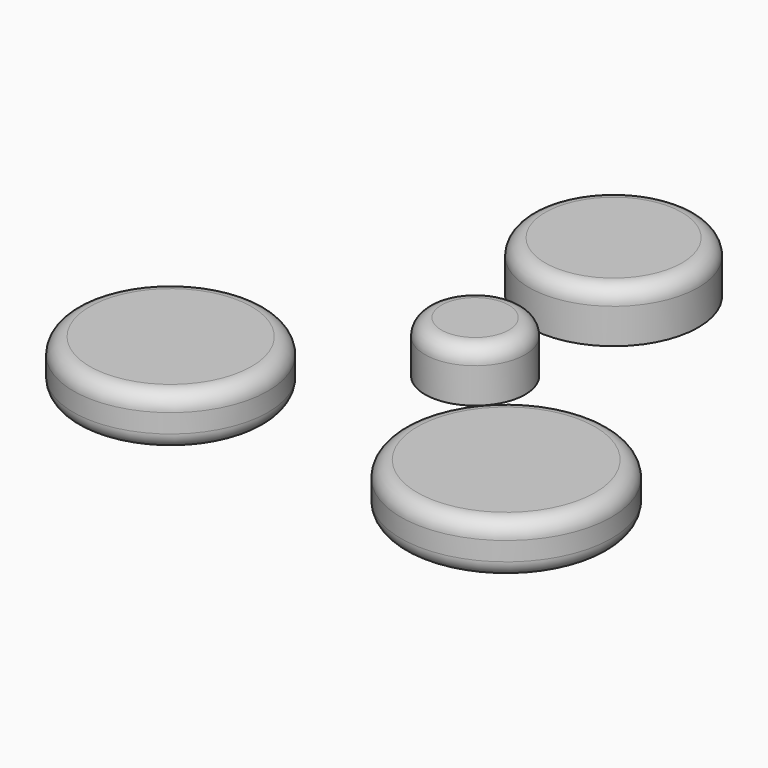
from build123d import *

# Parameters (mm, degrees)
F1_R     = 32.7456463168
F2_DEPTH = 15.9970168024
F1_R_2   = 30.2415831597
F1_R_3   = 26.3371113364
F0_R     = 15.5625582152
F3_R     = 5.08
F3_2_R   = 5.08
F3_3_R   = 5.08
F3_4_R   = 5.08


# Not quite as in the source:
# - a feature of the source that left no trace in its solid (it failed there, or was rolled back) is left out


with BuildPart() as f2:
    # F1 (on Top) → F2 (new body)
    with BuildSketch(Plane.XY):
        with Locations((52.5437146425, -53.609341383)):
            Circle(F1_R)
    extrude(amount=F2_DEPTH)

    # F3
    f3_edges = [f2.edges().sort_by_distance(p)[0] for p in [
        (19.798068, -53.609341, 15.997017),
        (19.798068, -53.609341, 0),
    ]]
    fillet(f3_edges, radius=F3_R)


with BuildPart() as f2b:
    # F1 (on Top) → F2, piece 2 (new body)
    with BuildSketch(Plane.XY):
        with Locations((-51.4770336449, -53.9423078299)):
            Circle(F1_R_2)
    extrude(amount=F2_DEPTH)

    # F3#2
    f3_2_edges = [f2b.edges().sort_by_distance(p)[0] for p in [
        (-81.718617, -53.942308, 15.997017),
        (-81.718617, -53.942308, 0),
    ]]
    fillet(f3_2_edges, radius=F3_2_R)


with BuildPart() as f2c:
    # F1 (on Top) → F2, piece 3 (new body)
    with BuildSketch(Plane.XY):
        with Locations((0, 53.7974014878)):
            Circle(F1_R_3)
    extrude(amount=F2_DEPTH)

    # F3#3
    f3_3_edges = [f2c.edges().sort_by_distance(p)[0] for p in [
        (-26.337111, 53.797401, 15.997017),
    ]]
    fillet(f3_3_edges, radius=F3_3_R)


with BuildPart() as f2d:
    # F0 (on Top) → F2, piece 4 (new body)
    with BuildSketch(Plane.XY):
        Circle(F0_R)
    extrude(amount=F2_DEPTH)

    # F3#4
    f3_4_edges = [f2d.edges().sort_by_distance(p)[0] for p in [
        (-15.562558, 0, 15.997017),
    ]]
    fillet(f3_4_edges, radius=F3_4_R)


solid = Compound([f2.part, f2b.part, f2c.part, f2d.part])
